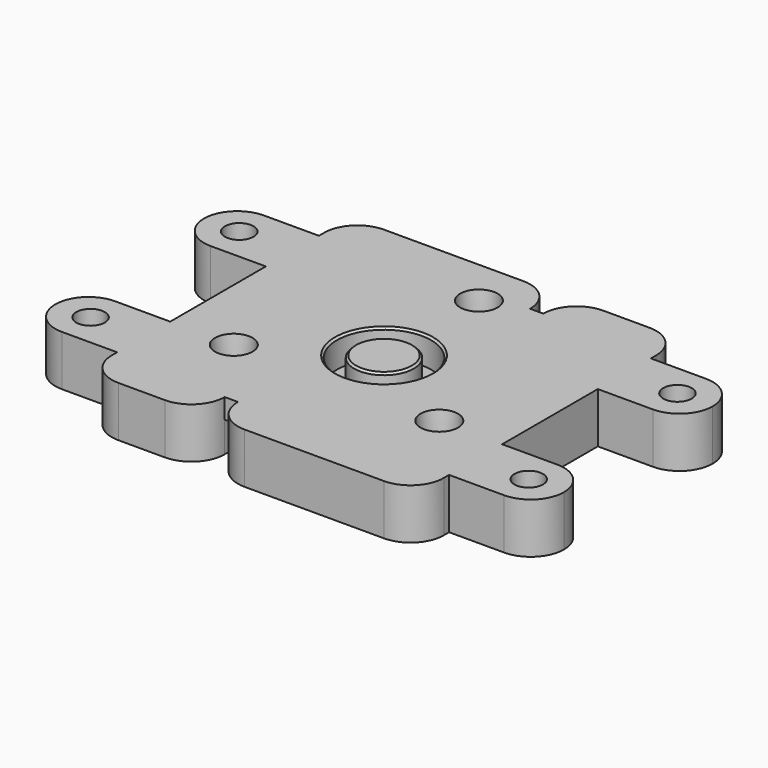
from build123d import *

# Parameters (mm, degrees)
F0_R        = 1.8
F0_W        = 13.3
F0_H        = 10
F0_R_2      = 2.15
F1_DEPTH    = 7.9
F2_R        = 2.575
F2_R_2      = 5.5
F2_W        = 13.3
F2_H        = 10
F2_R_3      = 2.15
F3_DEPTH    = 4.7
F4_T1_DEPTH = 4.7
F5_T1_DEPTH = 37.6
F6_SIZE     = 0.6
F7_SIZE2    = 0.25
F7_SIZE     = 3.7
F7_2_SIZE2  = 0.25
F7_2_SIZE   = 3.7
F7_3_SIZE2  = 0.25
F7_3_SIZE   = 3.7
F8_DEPTH    = 5
F9_R        = 7.1
F9_R_2      = 5.5
F10_DEPTH   = 4.2
F9_R_3      = 4.5
F11_DEPTH   = 4.2
F12_SIZE    = 0.3
F12_2_SIZE  = 0.3
F13_R       = 5.5
F13_R_2     = 2.1
F14_DEPTH   = 0.3
F16_DEPTH   = 3


# Not quite as in the source:
# - a fillet or chamfer that OpenCascade refuses, or shapes differently, is made with other operations: its cross-section is extruded or revolved along the edge and cut away or added


with BuildPart() as f1:
    # F0 (on Top) → F1 (new body)
    with BuildSketch(Plane.XY):
        Polygon((-10.5, 10.5), (6, 10.5), (6, 25), (-25, 25), (-25, 19), (-25, 9), (-25, -9), (-25, -19), (-25, -25), (-8, -25), (-8, -10.5), (-10.5, -10.5), align=None)
        with Locations((-15.475, -8.9344954157)):
            Circle(F0_R, mode=Mode.SUBTRACT)
        with Locations((0, 17.8689908314)):
            Circle(F0_R, mode=Mode.SUBTRACT)
        with Locations((-31.65, 14)):
            Rectangle(F0_W, F0_H)
        with Locations((-33, 14)):
            Circle(F0_R_2, mode=Mode.SUBTRACT)
        with Locations((-31.65, -14)):
            Rectangle(F0_W, F0_H)
        with Locations((-33, -14)):
            Circle(F0_R_2, mode=Mode.SUBTRACT)
    extrude(amount=F1_DEPTH)



with BuildPart() as f1b:
    # F0 (on Top) → F1, piece 2 (new body)
    with BuildSketch(Plane.XY):
        Polygon((8, 10.5), (10.5, 10.5), (10.5, -10.5), (-6, -10.5), (-6, -25), (25, -25), (25, -19), (25, -9), (25, 9), (25, 19), (25, 25), (8, 25), align=None)
        with Locations((15.475, -8.9344954157)):
            Circle(F0_R, mode=Mode.SUBTRACT)
        with Locations((31.65, -14)):
            Rectangle(F0_W, F0_H)
        with Locations((33, -14)):
            Circle(F0_R_2, mode=Mode.SUBTRACT)
        with Locations((31.65, 14)):
            Rectangle(F0_W, F0_H)
        with Locations((33, 14)):
            Circle(F0_R_2, mode=Mode.SUBTRACT)
    extrude(amount=F1_DEPTH)


with BuildPart() as f1_1:
    add(f1.part)

    add(f1b.part)  # F3 merges F1b
    # F2 (on face) → F3 (join)
    with BuildSketch(Plane.XY.offset(7.9)):
        Polygon((6, 10.5), (6, 25), (-25, 25), (-25, 19), (-25, 9), (-25, -9), (-25, -19), (-25, -25), (-8, -25), (-8, -10.5), (-10.5, -10.5), (-10.5, 10.5), align=None)
        with Locations((-15.475, -8.9344954157)):
            Circle(F2_R, mode=Mode.SUBTRACT)
        with Locations((0, 17.8689908314)):
            Circle(F2_R, mode=Mode.SUBTRACT)
        Polygon((25, 19), (25, 25), (8, 25), (8, 10.5), (8, 5), (6, 5), (6, 10.5), (-10.5, 10.5), (-10.5, -10.5), (-8, -10.5), (-8, -5), (-6, -5), (-6, -10.5), (-6, -25), (25, -25), (25, -19), (25, -9), (25, 9), align=None)
        with Locations((15.475, -8.9344954157)):
            Circle(F2_R, mode=Mode.SUBTRACT)
        Circle(F2_R_2, mode=Mode.SUBTRACT)
        with Locations((-31.65, -14)):
            Rectangle(F2_W, F2_H)
        with Locations((-33, -14)):
            Circle(F2_R_3, mode=Mode.SUBTRACT)
        with Locations((-31.65, 14)):
            Rectangle(F2_W, F2_H)
        with Locations((-33, 14)):
            Circle(F2_R_3, mode=Mode.SUBTRACT)
        with Locations((31.65, 14)):
            Rectangle(F2_W, F2_H)
        with Locations((33, 14)):
            Circle(F2_R_3, mode=Mode.SUBTRACT)
        with Locations((31.65, -14)):
            Rectangle(F2_W, F2_H)
        with Locations((33, -14)):
            Circle(F2_R_3, mode=Mode.SUBTRACT)
    extrude(amount=F3_DEPTH)

    # F4: fillet of radius 1 on 4 edges, made by hand

    # F4_s2 → F4_t1 (join)
    with BuildSketch(Plane.XY.offset(7.9)):
        with BuildLine():
            ThreePointArc((-7, -5), (-6.2928932188, -5.2928932188), (-6, -6))
            Line((-6, -6), (-6, -5))
            Line((-6, -5), (-7, -5))
        make_face()
        with BuildLine():
            ThreePointArc((-8, -6), (-7.7071067812, -5.2928932188), (-7, -5))
            Line((-7, -5), (-8, -5))
            Line((-8, -5), (-8, -6))
        make_face()
        with BuildLine():
            ThreePointArc((6, 6), (6.2928932188, 5.2928932188), (7, 5))
            Line((7, 5), (6, 5))
            Line((6, 5), (6, 6))
        make_face()
        with BuildLine():
            ThreePointArc((7, 5), (7.7071067812, 5.2928932188), (8, 6))
            Line((8, 6), (8, 5))
            Line((8, 5), (7, 5))
        make_face()
    extrude(amount=F4_T1_DEPTH)

    # F5: fillet of radius 5 on 16 edges, made by hand

    # F5_s2 → F5_t1 (cut)
    with BuildSketch(Plane.XY.offset(-12.5)):
        with BuildLine():
            ThreePointArc((-38.3, 14), (-36.8355339059, 10.4644660941), (-33.3, 9))
            Line((-33.3, 9), (-38.3, 9))
            Line((-38.3, 9), (-38.3, 14))
        make_face()
        with BuildLine():
            ThreePointArc((-33.3, 19), (-36.8355339059, 17.5355339059), (-38.3, 14))
            Line((-38.3, 14), (-38.3, 19))
            Line((-38.3, 19), (-33.3, 19))
        make_face()
        with BuildLine():
            ThreePointArc((-38.3, -14), (-36.8355339059, -17.5355339059), (-33.3, -19))
            Line((-33.3, -19), (-38.3, -19))
            Line((-38.3, -19), (-38.3, -14))
        make_face()
        with BuildLine():
            ThreePointArc((-33.3, -9), (-36.8355339059, -10.4644660941), (-38.3, -14))
            Line((-38.3, -14), (-38.3, -9))
            Line((-38.3, -9), (-33.3, -9))
        make_face()
        with BuildLine():
            ThreePointArc((33.3, -19), (36.8355339059, -17.5355339059), (38.3, -14))
            Line((38.3, -14), (38.3, -19))
            Line((38.3, -19), (33.3, -19))
        make_face()
        with BuildLine():
            ThreePointArc((38.3, -14), (36.8355339059, -10.4644660941), (33.3, -9))
            Line((33.3, -9), (38.3, -9))
            Line((38.3, -9), (38.3, -14))
        make_face()
        with BuildLine():
            ThreePointArc((33.3, 9), (36.8355339059, 10.4644660941), (38.3, 14))
            Line((38.3, 14), (38.3, 9))
            Line((38.3, 9), (33.3, 9))
        make_face()
        with BuildLine():
            ThreePointArc((38.3, 14), (36.8355339059, 17.5355339059), (33.3, 19))
            Line((33.3, 19), (38.3, 19))
            Line((38.3, 19), (38.3, 14))
        make_face()
        with BuildLine():
            ThreePointArc((-25, -20), (-23.5355339059, -23.5355339059), (-20, -25))
            Line((-20, -25), (-25, -25))
            Line((-25, -25), (-25, -20))
        make_face()
        with BuildLine():
            ThreePointArc((20, -25), (23.5355339059, -23.5355339059), (25, -20))
            Line((25, -20), (25, -25))
            Line((25, -25), (20, -25))
        make_face()
        with BuildLine():
            ThreePointArc((20, 25), (23.5355339059, 23.5355339059), (25, 20))
            Line((25, 20), (25, 25))
            Line((25, 25), (20, 25))
        make_face()
        with BuildLine():
            ThreePointArc((-20, 25), (-23.5355339059, 23.5355339059), (-25, 20))
            Line((-25, 20), (-25, 25))
            Line((-25, 25), (-20, 25))
        make_face()
        with BuildLine():
            ThreePointArc((6, 20), (4.5355339059, 23.5355339059), (1, 25))
            Line((1, 25), (6, 25))
            Line((6, 25), (6, 20))
        make_face()
        with BuildLine():
            ThreePointArc((8, 20), (9.4644660941, 23.5355339059), (13, 25))
            Line((13, 25), (8, 25))
            Line((8, 25), (8, 20))
        make_face()
        with BuildLine():
            ThreePointArc((-8, -20), (-9.4644660941, -23.5355339059), (-13, -25))
            Line((-13, -25), (-8, -25))
            Line((-8, -25), (-8, -20))
        make_face()
        with BuildLine():
            ThreePointArc((-6, -20), (-4.5355339059, -23.5355339059), (-1, -25))
            Line((-1, -25), (-6, -25))
            Line((-6, -25), (-6, -20))
        make_face()
    extrude(amount=F5_T1_DEPTH, mode=Mode.SUBTRACT)

    # F6
    f6_edges = [f1_1.edges().sort_by_distance(p)[0] for p in [
        (-10.5, 0, 0),
        (-9.25, -10.5, 0),
        (2.25, -10.5, 0),
        (10.5, 0, 0),
        (9.25, 10.5, 0),
        (-2.25, 10.5, 0),
        (-6, -8.25, 7.9),
        (8, 8.25, 7.9),
        (-8, -10.5, 3.95),
        (-6, -10.5, 3.95),
        (6, 10.5, 3.95),
        (8, 10.5, 3.95),
        (7.707107, 5.292893, 7.9),
        (6.292893, 5.292893, 7.9),
        (6, 8.25, 7.9),
        (-8, -8.25, 7.9),
        (-7.707107, -5.292893, 7.9),
        (-6.292893, -5.292893, 7.9),
    ]]
    chamfer(f6_edges, length=F6_SIZE)

    # F7
    f7_edges = [f1_1.edges().sort_by_distance(p)[0] for p in [
        (-2.575, 17.868991, 12.6),
    ]]
    f7_side = f1_1.faces().sort_by_distance((-2.575, 17.868991, 10.25))[0]
    chamfer(f7_edges, length=F7_SIZE, length2=F7_SIZE2, reference=f7_side)

    # F7#2
    f7_2_edges = [f1_1.edges().sort_by_distance(p)[0] for p in [
        (12.9, -8.934495, 12.6),
    ]]
    f7_2_side = f1_1.faces().sort_by_distance((12.9, -8.934495, 10.25))[0]
    chamfer(f7_2_edges, length=F7_2_SIZE, length2=F7_2_SIZE2, reference=f7_2_side)

    # F7#3
    f7_3_edges = [f1_1.edges().sort_by_distance(p)[0] for p in [
        (-18.05, -8.934495, 12.6),
    ]]
    f7_3_side = f1_1.faces().sort_by_distance((-18.05, -8.934495, 10.25))[0]
    chamfer(f7_3_edges, length=F7_3_SIZE, length2=F7_3_SIZE2, reference=f7_3_side)

    # F0 (on Top) → F8 (cut)
    with BuildSketch(Plane.XY):
        Polygon((-10.5, 10.5), (6, 10.5), (6, 25), (-25, 25), (-25, 19), (-25, 9), (-25, -9), (-25, -19), (-25, -25), (-8, -25), (-8, -10.5), (-10.5, -10.5), align=None)
        with Locations((-15.475, -8.9344954157)):
            Circle(F0_R, mode=Mode.SUBTRACT)
        with Locations((0, 17.8689908314)):
            Circle(F0_R, mode=Mode.SUBTRACT)
        Polygon((8, 10.5), (10.5, 10.5), (10.5, -10.5), (-6, -10.5), (-6, -25), (25, -25), (25, -19), (25, -9), (25, 9), (25, 19), (25, 25), (8, 25), align=None)
        with Locations((15.475, -8.9344954157)):
            Circle(F0_R, mode=Mode.SUBTRACT)
        with Locations((-31.65, -14)):
            Rectangle(F0_W, F0_H)
        with Locations((-33, -14)):
            Circle(F0_R_2, mode=Mode.SUBTRACT)
        with Locations((-31.65, 14)):
            Rectangle(F0_W, F0_H)
        with Locations((-33, 14)):
            Circle(F0_R_2, mode=Mode.SUBTRACT)
        with Locations((31.65, 14)):
            Rectangle(F0_W, F0_H)
        with Locations((33, 14)):
            Circle(F0_R_2, mode=Mode.SUBTRACT)
        with Locations((31.65, -14)):
            Rectangle(F0_W, F0_H)
        with Locations((33, -14)):
            Circle(F0_R_2, mode=Mode.SUBTRACT)
    extrude(amount=F8_DEPTH, mode=Mode.SUBTRACT)

    # F9 (on face) → F10 (cut)
    with BuildSketch(Plane.XY.offset(12.6)):
        Circle(F9_R)
        Circle(F9_R_2, mode=Mode.SUBTRACT)
    extrude(amount=-F10_DEPTH, mode=Mode.SUBTRACT)

    # F12
    f12_edges = [f1_1.edges().sort_by_distance(p)[0] for p in [
        (-5.5, 0, 7.9),
        (-7.1, 0, 12.6),
    ]]
    chamfer(f12_edges, length=F12_SIZE)



with BuildPart() as f11:
    # F9 (on face) → F11 (new body, through all)
    with BuildSketch(Plane.XY.offset(12.6)):
        Circle(F9_R_3)
    extrude(amount=-F11_DEPTH)

    # F12#2
    f12_2_edges = [f11.edges().sort_by_distance(p)[0] for p in [
        (-4.5, 0, 12.6),
    ]]
    chamfer(f12_2_edges, length=F12_2_SIZE)


with BuildPart() as f1_2:
    add(f1_1.part)

    add(f11.part)  # F14 merges F11
    # F13 (on face) → F14 (join)
    with BuildSketch(Plane.XY.offset(8.4)):
        Circle(F13_R)
        Circle(F13_R_2, mode=Mode.SUBTRACT)
    extrude(amount=-F14_DEPTH)

    # F15 (on face) → F16 (join)
    with BuildSketch(Plane.XY.offset(12.6)):
        with BuildLine():
            Line((-6, -20), (-6, -6))
            ThreePointArc((-6, -6), (-6.2928932188, -5.2928932188), (-7, -5))
            ThreePointArc((-7, -5), (-7.7071067812, -5.2928932188), (-8, -6))
            Line((-8, -6), (-8, -20))
            Line((-8, -20), (-6, -20))
        make_face()
        with BuildLine():
            Line((8, 6), (8, 20))
            Line((8, 20), (6, 20))
            Line((6, 20), (6, 11.1))
            Line((6, 11.1), (6, 6))
            ThreePointArc((6, 6), (6.2928932188, 5.2928932188), (7, 5))
            ThreePointArc((7, 5), (7.7071067812, 5.2928932188), (8, 6))
        make_face()
    extrude(amount=-F16_DEPTH)


solid = f1_2.part
